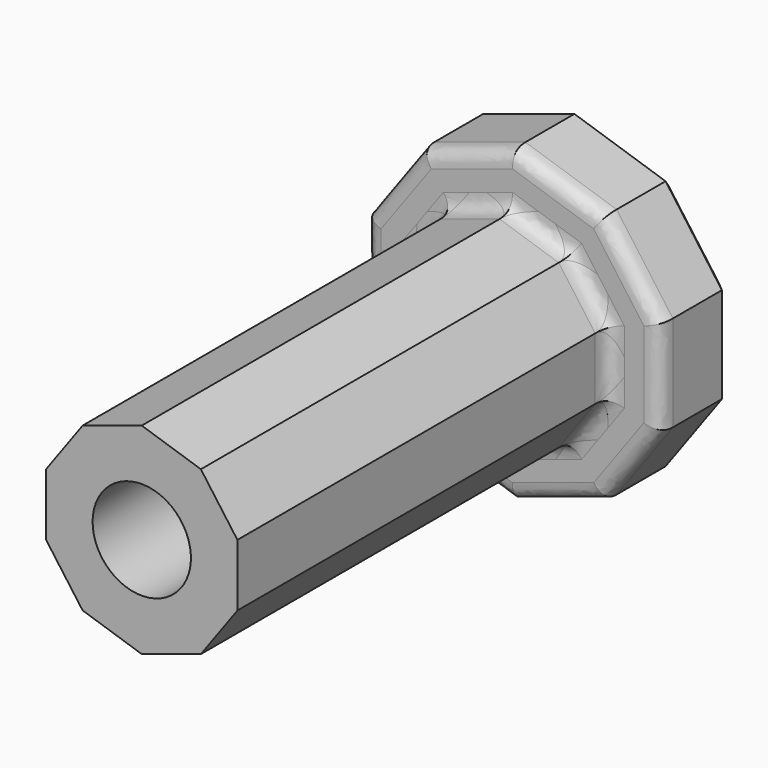
from build123d import *

# Parameters (mm, degrees)
F1_DEPTH      = 76.2
F3_DEPTH      = 6.985
F4_T4_DEPTH   = 21.3495807372
F4_T10_DEPTH  = 21.3495807372
F4_T16_DEPTH  = 21.3495807372
F4_T22_DEPTH  = 21.3495807372
F4_T28_DEPTH  = 21.3495807372
F4_T34_DEPTH  = 21.3495807372
F4_T40_DEPTH  = 21.3495807372
F4_T46_DEPTH  = 21.3495807372
F4_T52_DEPTH  = 21.3495807372
F4_T58_DEPTH  = 21.3495807372
F4_T65_DEPTH  = 21.3495807372
F4_T69_DEPTH  = 21.3495807372
F4_T76_DEPTH  = 21.3495807372
F4_T80_DEPTH  = 21.3495807372
F4_T87_DEPTH  = 21.3495807372
F4_T91_DEPTH  = 21.3495807372
F4_T98_DEPTH  = 21.3495807372
F4_T102_DEPTH = 21.3495807372
F4_T109_DEPTH = 21.3495807372
F4_T113_DEPTH = 21.3495807372
F4_T120_DEPTH = 21.3495807372
F4_T124_DEPTH = 21.3495807372
F4_T131_DEPTH = 21.3495807372
F4_T135_DEPTH = 21.3495807372
F4_T142_DEPTH = 21.3495807372
F4_T146_DEPTH = 21.3495807372
F4_T153_DEPTH = 21.3495807372
F4_T157_DEPTH = 21.3495807372
F4_T164_DEPTH = 21.3495807372
F4_T168_DEPTH = 21.3495807372
F4_T171_DEPTH = 26.3812242456
F4_T173_DEPTH = 26.3812242456
F4_T175_DEPTH = 26.3812242456
F4_T177_DEPTH = 26.3812242456
F4_T179_DEPTH = 26.3812242456
F4_T181_DEPTH = 26.3812242456
F4_T183_DEPTH = 26.3812242456
F4_T185_DEPTH = 26.3812242456
F4_T187_DEPTH = 26.3812242456
F5_SIZE       = 2.413
F7_D          = 14.68374


# Not quite as in the source:
# - a fillet or chamfer that OpenCascade refuses, or shapes differently, is made with other operations: its cross-section is extruded or revolved along the edge and cut away or added


with BuildPart() as f1:
    # F0 (on Front) → F1 (new body)
    with BuildSketch(Plane.XZ):
        Polygon((-14.2875006422, 4.6422903686), (-14.2875006422, -4.6422903686), (-8.8301610112, -12.1536739707), (0, -15.0227672041), (8.8301610112, -12.1536739707), (14.2875006422, -4.6422903686), (14.2875006422, 4.6422903686), (8.8301610112, 12.1536739707), (0, 15.0227672041), (-8.8301610112, 12.1536739707), align=None)
    extrude(amount=F1_DEPTH)

    # F2 (on Front) → F3 (join, symmetric)
    with BuildSketch(Plane.XZ):
        Polygon((-22.0304038376, 7.1581121228), (-22.0304038376, -7.1581121228), (-13.6155383575, -18.7401808327), (0, -23.1641374199), (13.6155383575, -18.7401808327), (22.0304038376, -7.1581121228), (22.0304038376, 7.1581121228), (13.6155383575, 18.7401808327), (0, 23.1641374199), (-13.6155383575, 18.7401808327), align=None)
    extrude(amount=F3_DEPTH, both=True)

    # F4: fillet of radius 2.413 on 20 edges, made by hand


with BuildPart() as f4_tool2:
    # F4_s3 → F4_t4 (new body)
    with BuildSketch(Plane(origin=(10.1523289401, 0, 3.2986916353), x_dir=(0, 1, 0), z_dir=(-0.9510565163, 0, -0.3090169944))):
        with BuildLine():
            add(Edge.make_bspline(
                [(-9.398, -14.2875006422), (-6.985, -14.2875006422), (-6.985, -16.7005006422)],
                knots=[0, 0, 0, 1, 1, 1], degree=2, weights=[1, 1, 1]))
            Line((-6.985, -16.7005006422), (-6.985, -14.2875006422))
            Line((-6.985, -14.2875006422), (-9.398, -14.2875006422))
        make_face()
    extrude(amount=F4_T4_DEPTH)

    split(bisect_by=Plane(origin=(-11.5588308267, 0, 8.3979821696), x_dir=(0, 1, 0), z_dir=(0.8090169944, 0, -0.5877852523)), keep=Keep.TOP)

    split(bisect_by=Plane(origin=(4.4150805056, 0, 13.5882205874), x_dir=(0, 1, 0), z_dir=(-0.3090169944, 0, -0.9510565163)), keep=Keep.TOP)


with BuildPart() as f1_1:
    add(f1.part)

    # F4_t1: union F4_tool2
    add(f4_tool2.part)


with BuildPart() as f4_tool8:
    # F4_s9 → F4_t10 (new body)
    with BuildSketch(Plane(origin=(6.27448435, 0, 8.6360868196), x_dir=(0, 1, 0), z_dir=(-0.5877852523, 0, -0.8090169944))):
        with BuildLine():
            add(Edge.make_bspline(
                [(-6.985, -16.7005006422), (-6.985, -14.2875006422), (-9.398, -14.2875006422)],
                knots=[0, 0, 0, 1, 1, 1], degree=2, weights=[1, 1, 1]))
            Line((-9.398, -14.2875006422), (-6.985, -14.2875006422))
            Line((-6.985, -14.2875006422), (-6.985, -16.7005006422))
        make_face()
    extrude(amount=F4_T10_DEPTH)

    split(bisect_by=Plane(origin=(-4.4150805056, 0, 13.5882205874), x_dir=(0, 1, 0), z_dir=(0.3090169944, 0, -0.9510565163)), keep=Keep.TOP)

    split(bisect_by=Plane.YZ.offset(-14.2875006422), keep=Keep.TOP)


with BuildPart() as f1_2:
    add(f1_1.part)

    # F4_t7: union F4_tool8
    add(f4_tool8.part)


with BuildPart() as f4_tool14:
    # F4_s15 → F4_t16 (new body)
    with BuildSketch(Plane.XY.offset(10.6747903686)):
        with BuildLine():
            add(Edge.make_bspline(
                [(-16.7005006422, -6.985), (-14.2875006422, -6.985), (-14.2875006422, -9.398)],
                knots=[0, 0, 0, 1, 1, 1], degree=2, weights=[1, 1, 1]))
            Line((-14.2875006422, -9.398), (-14.2875006422, -6.985))
            Line((-14.2875006422, -6.985), (-16.7005006422, -6.985))
        make_face()
    extrude(amount=-F4_T16_DEPTH)

    split(bisect_by=Plane(origin=(-11.5588308267, 0, 8.3979821696), x_dir=(0, 1, 0), z_dir=(0.8090169944, 0, -0.5877852523)), keep=Keep.TOP)

    split(bisect_by=Plane(origin=(-11.5588308267, 0, -8.3979821696), x_dir=(0, 1, 0), z_dir=(0.8090169944, 0, 0.5877852523)), keep=Keep.TOP)


with BuildPart() as f1_3:
    add(f1_2.part)

    # F4_t13: union F4_tool14
    add(f4_tool14.part)


with BuildPart() as f4_tool20:
    # F4_s21 → F4_t22 (new body)
    with BuildSketch(Plane(origin=(-6.27448435, 0, 8.6360868196), x_dir=(0, 1, 0), z_dir=(0.5877852523, 0, -0.8090169944))):
        with BuildLine():
            add(Edge.make_bspline(
                [(-6.985, -16.7005006422), (-6.985, -14.2875006422), (-9.398, -14.2875006422)],
                knots=[0, 0, 0, 1, 1, 1], degree=2, weights=[1, 1, 1]))
            Line((-9.398, -14.2875006422), (-6.985, -14.2875006422))
            Line((-6.985, -14.2875006422), (-6.985, -16.7005006422))
        make_face()
    extrude(amount=F4_T22_DEPTH)

    split(bisect_by=Plane.YZ.offset(-14.2875006422), keep=Keep.TOP)

    split(bisect_by=Plane(origin=(-4.4150805056, 0, -13.5882205874), x_dir=(0, 1, 0), z_dir=(0.3090169944, 0, 0.9510565163)), keep=Keep.TOP)


with BuildPart() as f1_4:
    add(f1_3.part)

    # F4_t19: union F4_tool20
    add(f4_tool20.part)


with BuildPart() as f4_tool26:
    # F4_s27 → F4_t28 (new body)
    with BuildSketch(Plane(origin=(-10.1523289401, 0, 3.2986916353), x_dir=(0, 1, 0), z_dir=(0.9510565163, 0, -0.3090169944))):
        with BuildLine():
            add(Edge.make_bspline(
                [(-6.985, -16.7005006422), (-6.985, -14.2875006422), (-9.398, -14.2875006422)],
                knots=[0, 0, 0, 1, 1, 1], degree=2, weights=[1, 1, 1]))
            Line((-9.398, -14.2875006422), (-6.985, -14.2875006422))
            Line((-6.985, -14.2875006422), (-6.985, -16.7005006422))
        make_face()
    extrude(amount=F4_T28_DEPTH)

    split(bisect_by=Plane(origin=(-11.5588308267, 0, -8.3979821696), x_dir=(0, 1, 0), z_dir=(0.8090169944, 0, 0.5877852523)), keep=Keep.TOP)

    split(bisect_by=Plane(origin=(4.4150805056, 0, -13.5882205874), x_dir=(0, 1, 0), z_dir=(-0.3090169944, 0, 0.9510565163)), keep=Keep.TOP)


with BuildPart() as f1_5:
    add(f1_4.part)

    # F4_t25: union F4_tool26
    add(f4_tool26.part)


with BuildPart() as f4_tool32:
    # F4_s33 → F4_t34 (new body)
    with BuildSketch(Plane(origin=(-10.1523289401, 0, -3.2986916353), x_dir=(0, 1, 0), z_dir=(0.9510565163, 0, 0.3090169944))):
        with BuildLine():
            add(Edge.make_bspline(
                [(-6.985, -16.7005006422), (-6.985, -14.2875006422), (-9.398, -14.2875006422)],
                knots=[0, 0, 0, 1, 1, 1], degree=2, weights=[1, 1, 1]))
            Line((-9.398, -14.2875006422), (-6.985, -14.2875006422))
            Line((-6.985, -14.2875006422), (-6.985, -16.7005006422))
        make_face()
    extrude(amount=F4_T34_DEPTH)

    split(bisect_by=Plane(origin=(-4.4150805056, 0, -13.5882205874), x_dir=(0, 1, 0), z_dir=(0.3090169944, 0, 0.9510565163)), keep=Keep.TOP)

    split(bisect_by=Plane(origin=(11.5588308267, 0, -8.3979821696), x_dir=(0, 1, 0), z_dir=(-0.8090169944, 0, 0.5877852523)), keep=Keep.TOP)


with BuildPart() as f1_6:
    add(f1_5.part)

    # F4_t31: union F4_tool32
    add(f4_tool32.part)


with BuildPart() as f4_tool38:
    # F4_s39 → F4_t40 (new body)
    with BuildSketch(Plane(origin=(-6.27448435, 0, -8.6360868196), x_dir=(0, 1, 0), z_dir=(0.5877852523, 0, 0.8090169944))):
        with BuildLine():
            add(Edge.make_bspline(
                [(-6.985, -16.7005006422), (-6.985, -14.2875006422), (-9.398, -14.2875006422)],
                knots=[0, 0, 0, 1, 1, 1], degree=2, weights=[1, 1, 1]))
            Line((-9.398, -14.2875006422), (-6.985, -14.2875006422))
            Line((-6.985, -14.2875006422), (-6.985, -16.7005006422))
        make_face()
    extrude(amount=F4_T40_DEPTH)

    split(bisect_by=Plane(origin=(4.4150805056, 0, -13.5882205874), x_dir=(0, 1, 0), z_dir=(-0.3090169944, 0, 0.9510565163)), keep=Keep.TOP)

    split(bisect_by=Plane.YZ.offset(14.2875006422), keep=Keep.BOTTOM)


with BuildPart() as f1_7:
    add(f1_6.part)

    # F4_t37: union F4_tool38
    add(f4_tool38.part)


with BuildPart() as f4_tool44:
    # F4_s45 → F4_t46 (new body)
    with BuildSketch(Plane.XY.offset(-10.6747903686)):
        with BuildLine():
            add(Edge.make_bspline(
                [(16.7005006422, -6.985), (14.2875006422, -6.985), (14.2875006422, -9.398)],
                knots=[0, 0, 0, 1, 1, 1], degree=2, weights=[1, 1, 1]))
            Line((14.2875006422, -9.398), (14.2875006422, -6.985))
            Line((14.2875006422, -6.985), (16.7005006422, -6.985))
        make_face()
    extrude(amount=F4_T46_DEPTH)

    split(bisect_by=Plane(origin=(11.5588308267, 0, -8.3979821696), x_dir=(0, 1, 0), z_dir=(-0.8090169944, 0, 0.5877852523)), keep=Keep.TOP)

    split(bisect_by=Plane(origin=(11.5588308267, 0, 8.3979821696), x_dir=(0, 1, 0), z_dir=(-0.8090169944, 0, -0.5877852523)), keep=Keep.TOP)


with BuildPart() as f1_8:
    add(f1_7.part)

    # F4_t43: union F4_tool44
    add(f4_tool44.part)


with BuildPart() as f4_tool50:
    # F4_s51 → F4_t52 (new body)
    with BuildSketch(Plane(origin=(6.27448435, 0, -8.6360868196), x_dir=(0, 1, 0), z_dir=(-0.5877852523, 0, 0.8090169944))):
        with BuildLine():
            add(Edge.make_bspline(
                [(-6.985, -16.7005006422), (-6.985, -14.2875006422), (-9.398, -14.2875006422)],
                knots=[0, 0, 0, 1, 1, 1], degree=2, weights=[1, 1, 1]))
            Line((-9.398, -14.2875006422), (-6.985, -14.2875006422))
            Line((-6.985, -14.2875006422), (-6.985, -16.7005006422))
        make_face()
    extrude(amount=F4_T52_DEPTH)

    split(bisect_by=Plane(origin=(4.4150805056, 0, 13.5882205874), x_dir=(0, 1, 0), z_dir=(-0.3090169944, 0, -0.9510565163)), keep=Keep.TOP)

    split(bisect_by=Plane.YZ.offset(14.2875006422), keep=Keep.BOTTOM)


with BuildPart() as f1_9:
    add(f1_8.part)

    # F4_t49: union F4_tool50
    add(f4_tool50.part)


with BuildPart() as f4_tool56:
    # F4_s57 → F4_t58 (new body)
    with BuildSketch(Plane(origin=(10.1523289401, 0, -3.2986916353), x_dir=(0, 1, 0), z_dir=(-0.9510565163, 0, 0.3090169944))):
        with BuildLine():
            add(Edge.make_bspline(
                [(-6.985, -16.7005006422), (-6.985, -14.2875006422), (-9.398, -14.2875006422)],
                knots=[0, 0, 0, 1, 1, 1], degree=2, weights=[1, 1, 1]))
            Line((-9.398, -14.2875006422), (-6.985, -14.2875006422))
            Line((-6.985, -14.2875006422), (-6.985, -16.7005006422))
        make_face()
    extrude(amount=F4_T58_DEPTH)

    split(bisect_by=Plane(origin=(-4.4150805056, 0, 13.5882205874), x_dir=(0, 1, 0), z_dir=(0.3090169944, 0, -0.9510565163)), keep=Keep.TOP)

    split(bisect_by=Plane(origin=(11.5588308267, 0, 8.3979821696), x_dir=(0, 1, 0), z_dir=(-0.8090169944, 0, -0.5877852523)), keep=Keep.TOP)


with BuildPart() as f1_10:
    add(f1_9.part)

    # F4_t55: union F4_tool56
    add(f4_tool56.part)


with BuildPart() as f4_tool63:
    # F4_s64 → F4_t65 (new body)
    with BuildSketch(Plane(origin=(10.1523289401, 0, 3.2986916353), x_dir=(0, 1, 0), z_dir=(-0.9510565163, 0, -0.3090169944))):
        with BuildLine():
            add(Edge.make_bspline(
                [(-9.398, -14.2875006422), (-6.985, -14.2875006422), (-6.985, -16.7005006422)],
                knots=[0, 0, 0, 1, 1, 1], degree=2, weights=[1, 1, 1]))
            Line((-6.985, -16.7005006422), (-6.985, -14.2875006422))
            Line((-6.985, -14.2875006422), (-9.398, -14.2875006422))
        make_face()
    extrude(amount=F4_T65_DEPTH)

    split(bisect_by=Plane(origin=(4.4150805056, 0, 13.5882205874), x_dir=(0, 1, 0), z_dir=(0.3090169944, 0, 0.9510565163)), keep=Keep.TOP)


with BuildPart() as f4_tool67:
    # F4_s68 → F4_t69 (new body)
    with BuildSketch(Plane(origin=(10.1523289401, 0, -3.2986916353), x_dir=(0, 1, 0), z_dir=(-0.9510565163, 0, 0.3090169944))):
        with BuildLine():
            add(Edge.make_bspline(
                [(-6.985, -16.7005006422), (-6.985, -14.2875006422), (-9.398, -14.2875006422)],
                knots=[0, 0, 0, 1, 1, 1], degree=2, weights=[1, 1, 1]))
            Line((-9.398, -14.2875006422), (-6.985, -14.2875006422))
            Line((-6.985, -14.2875006422), (-6.985, -16.7005006422))
        make_face()
    extrude(amount=F4_T69_DEPTH)

    split(bisect_by=Plane(origin=(-4.4150805056, 0, 13.5882205874), x_dir=(0, 1, 0), z_dir=(-0.3090169944, 0, 0.9510565163)), keep=Keep.TOP)


with BuildPart() as f4_tool63_1:
    add(f4_tool63.part)

    # F4_t71: intersect F4_tool67
    add(f4_tool67.part, mode=Mode.INTERSECT)


with BuildPart() as f1_11:
    add(f1_10.part)

    # F4_t61: union F4_tool63
    add(f4_tool63_1.part)


with BuildPart() as f4_tool74:
    # F4_s75 → F4_t76 (new body)
    with BuildSketch(Plane(origin=(10.1523289401, 0, 3.2986916353), x_dir=(0, 1, 0), z_dir=(-0.9510565163, 0, -0.3090169944))):
        with BuildLine():
            add(Edge.make_bspline(
                [(-9.398, -14.2875006422), (-6.985, -14.2875006422), (-6.985, -16.7005006422)],
                knots=[0, 0, 0, 1, 1, 1], degree=2, weights=[1, 1, 1]))
            Line((-6.985, -16.7005006422), (-6.985, -14.2875006422))
            Line((-6.985, -14.2875006422), (-9.398, -14.2875006422))
        make_face()
    extrude(amount=F4_T76_DEPTH)

    split(bisect_by=Plane(origin=(-11.5588308267, 0, 8.3979821696), x_dir=(0, 1, 0), z_dir=(-0.8090169944, 0, 0.5877852523)), keep=Keep.TOP)


with BuildPart() as f4_tool78:
    # F4_s79 → F4_t80 (new body)
    with BuildSketch(Plane(origin=(6.27448435, 0, 8.6360868196), x_dir=(0, 1, 0), z_dir=(-0.5877852523, 0, -0.8090169944))):
        with BuildLine():
            add(Edge.make_bspline(
                [(-6.985, -16.7005006422), (-6.985, -14.2875006422), (-9.398, -14.2875006422)],
                knots=[0, 0, 0, 1, 1, 1], degree=2, weights=[1, 1, 1]))
            Line((-9.398, -14.2875006422), (-6.985, -14.2875006422))
            Line((-6.985, -14.2875006422), (-6.985, -16.7005006422))
        make_face()
    extrude(amount=F4_T80_DEPTH)

    split(bisect_by=Plane(origin=(-4.4150805056, 0, 13.5882205874), x_dir=(0, 1, 0), z_dir=(-0.3090169944, 0, 0.9510565163)), keep=Keep.TOP)


with BuildPart() as f4_tool74_1:
    add(f4_tool74.part)

    # F4_t82: intersect F4_tool78
    add(f4_tool78.part, mode=Mode.INTERSECT)


with BuildPart() as f1_12:
    add(f1_11.part)

    # F4_t72: union F4_tool74
    add(f4_tool74_1.part)


with BuildPart() as f4_tool85:
    # F4_s86 → F4_t87 (new body)
    with BuildSketch(Plane(origin=(6.27448435, 0, 8.6360868196), x_dir=(0, 1, 0), z_dir=(-0.5877852523, 0, -0.8090169944))):
        with BuildLine():
            add(Edge.make_bspline(
                [(-6.985, -16.7005006422), (-6.985, -14.2875006422), (-9.398, -14.2875006422)],
                knots=[0, 0, 0, 1, 1, 1], degree=2, weights=[1, 1, 1]))
            Line((-9.398, -14.2875006422), (-6.985, -14.2875006422))
            Line((-6.985, -14.2875006422), (-6.985, -16.7005006422))
        make_face()
    extrude(amount=F4_T87_DEPTH)

    split(bisect_by=Plane.YZ.offset(-14.2875006422), keep=Keep.BOTTOM)


with BuildPart() as f4_tool89:
    # F4_s90 → F4_t91 (new body)
    with BuildSketch(Plane.XY.offset(10.6747903686)):
        with BuildLine():
            add(Edge.make_bspline(
                [(-16.7005006422, -6.985), (-14.2875006422, -6.985), (-14.2875006422, -9.398)],
                knots=[0, 0, 0, 1, 1, 1], degree=2, weights=[1, 1, 1]))
            Line((-14.2875006422, -9.398), (-14.2875006422, -6.985))
            Line((-14.2875006422, -6.985), (-16.7005006422, -6.985))
        make_face()
    extrude(amount=-F4_T91_DEPTH)

    split(bisect_by=Plane(origin=(-11.5588308267, 0, 8.3979821696), x_dir=(0, 1, 0), z_dir=(-0.8090169944, 0, 0.5877852523)), keep=Keep.TOP)


with BuildPart() as f4_tool85_1:
    add(f4_tool85.part)

    # F4_t93: intersect F4_tool89
    add(f4_tool89.part, mode=Mode.INTERSECT)


with BuildPart() as f1_13:
    add(f1_12.part)

    # F4_t83: union F4_tool85
    add(f4_tool85_1.part)


with BuildPart() as f4_tool96:
    # F4_s97 → F4_t98 (new body)
    with BuildSketch(Plane.XY.offset(10.6747903686)):
        with BuildLine():
            add(Edge.make_bspline(
                [(-16.7005006422, -6.985), (-14.2875006422, -6.985), (-14.2875006422, -9.398)],
                knots=[0, 0, 0, 1, 1, 1], degree=2, weights=[1, 1, 1]))
            Line((-14.2875006422, -9.398), (-14.2875006422, -6.985))
            Line((-14.2875006422, -6.985), (-16.7005006422, -6.985))
        make_face()
    extrude(amount=-F4_T98_DEPTH)

    split(bisect_by=Plane(origin=(-11.5588308267, 0, -8.3979821696), x_dir=(0, 1, 0), z_dir=(-0.8090169944, 0, -0.5877852523)), keep=Keep.TOP)


with BuildPart() as f4_tool100:
    # F4_s101 → F4_t102 (new body)
    with BuildSketch(Plane(origin=(-6.27448435, 0, 8.6360868196), x_dir=(0, 1, 0), z_dir=(0.5877852523, 0, -0.8090169944))):
        with BuildLine():
            add(Edge.make_bspline(
                [(-6.985, -16.7005006422), (-6.985, -14.2875006422), (-9.398, -14.2875006422)],
                knots=[0, 0, 0, 1, 1, 1], degree=2, weights=[1, 1, 1]))
            Line((-9.398, -14.2875006422), (-6.985, -14.2875006422))
            Line((-6.985, -14.2875006422), (-6.985, -16.7005006422))
        make_face()
    extrude(amount=F4_T102_DEPTH)

    split(bisect_by=Plane.YZ.offset(-14.2875006422), keep=Keep.BOTTOM)


with BuildPart() as f4_tool96_1:
    add(f4_tool96.part)

    # F4_t104: intersect F4_tool100
    add(f4_tool100.part, mode=Mode.INTERSECT)


with BuildPart() as f1_14:
    add(f1_13.part)

    # F4_t94: union F4_tool96
    add(f4_tool96_1.part)


with BuildPart() as f4_tool107:
    # F4_s108 → F4_t109 (new body)
    with BuildSketch(Plane(origin=(-6.27448435, 0, 8.6360868196), x_dir=(0, 1, 0), z_dir=(0.5877852523, 0, -0.8090169944))):
        with BuildLine():
            add(Edge.make_bspline(
                [(-6.985, -16.7005006422), (-6.985, -14.2875006422), (-9.398, -14.2875006422)],
                knots=[0, 0, 0, 1, 1, 1], degree=2, weights=[1, 1, 1]))
            Line((-9.398, -14.2875006422), (-6.985, -14.2875006422))
            Line((-6.985, -14.2875006422), (-6.985, -16.7005006422))
        make_face()
    extrude(amount=F4_T109_DEPTH)

    split(bisect_by=Plane(origin=(-4.4150805056, 0, -13.5882205874), x_dir=(0, 1, 0), z_dir=(-0.3090169944, 0, -0.9510565163)), keep=Keep.TOP)


with BuildPart() as f4_tool111:
    # F4_s112 → F4_t113 (new body)
    with BuildSketch(Plane(origin=(-10.1523289401, 0, 3.2986916353), x_dir=(0, 1, 0), z_dir=(0.9510565163, 0, -0.3090169944))):
        with BuildLine():
            add(Edge.make_bspline(
                [(-6.985, -16.7005006422), (-6.985, -14.2875006422), (-9.398, -14.2875006422)],
                knots=[0, 0, 0, 1, 1, 1], degree=2, weights=[1, 1, 1]))
            Line((-9.398, -14.2875006422), (-6.985, -14.2875006422))
            Line((-6.985, -14.2875006422), (-6.985, -16.7005006422))
        make_face()
    extrude(amount=F4_T113_DEPTH)

    split(bisect_by=Plane(origin=(-11.5588308267, 0, -8.3979821696), x_dir=(0, 1, 0), z_dir=(-0.8090169944, 0, -0.5877852523)), keep=Keep.TOP)


with BuildPart() as f4_tool107_1:
    add(f4_tool107.part)

    # F4_t115: intersect F4_tool111
    add(f4_tool111.part, mode=Mode.INTERSECT)


with BuildPart() as f1_15:
    add(f1_14.part)

    # F4_t105: union F4_tool107
    add(f4_tool107_1.part)


with BuildPart() as f4_tool118:
    # F4_s119 → F4_t120 (new body)
    with BuildSketch(Plane(origin=(-10.1523289401, 0, 3.2986916353), x_dir=(0, 1, 0), z_dir=(0.9510565163, 0, -0.3090169944))):
        with BuildLine():
            add(Edge.make_bspline(
                [(-6.985, -16.7005006422), (-6.985, -14.2875006422), (-9.398, -14.2875006422)],
                knots=[0, 0, 0, 1, 1, 1], degree=2, weights=[1, 1, 1]))
            Line((-9.398, -14.2875006422), (-6.985, -14.2875006422))
            Line((-6.985, -14.2875006422), (-6.985, -16.7005006422))
        make_face()
    extrude(amount=F4_T120_DEPTH)

    split(bisect_by=Plane(origin=(4.4150805056, 0, -13.5882205874), x_dir=(0, 1, 0), z_dir=(0.3090169944, 0, -0.9510565163)), keep=Keep.TOP)


with BuildPart() as f4_tool122:
    # F4_s123 → F4_t124 (new body)
    with BuildSketch(Plane(origin=(-10.1523289401, 0, -3.2986916353), x_dir=(0, 1, 0), z_dir=(0.9510565163, 0, 0.3090169944))):
        with BuildLine():
            add(Edge.make_bspline(
                [(-6.985, -16.7005006422), (-6.985, -14.2875006422), (-9.398, -14.2875006422)],
                knots=[0, 0, 0, 1, 1, 1], degree=2, weights=[1, 1, 1]))
            Line((-9.398, -14.2875006422), (-6.985, -14.2875006422))
            Line((-6.985, -14.2875006422), (-6.985, -16.7005006422))
        make_face()
    extrude(amount=F4_T124_DEPTH)

    split(bisect_by=Plane(origin=(-4.4150805056, 0, -13.5882205874), x_dir=(0, 1, 0), z_dir=(-0.3090169944, 0, -0.9510565163)), keep=Keep.TOP)


with BuildPart() as f4_tool118_1:
    add(f4_tool118.part)

    # F4_t126: intersect F4_tool122
    add(f4_tool122.part, mode=Mode.INTERSECT)


with BuildPart() as f1_16:
    add(f1_15.part)

    # F4_t116: union F4_tool118
    add(f4_tool118_1.part)


with BuildPart() as f4_tool129:
    # F4_s130 → F4_t131 (new body)
    with BuildSketch(Plane(origin=(-10.1523289401, 0, -3.2986916353), x_dir=(0, 1, 0), z_dir=(0.9510565163, 0, 0.3090169944))):
        with BuildLine():
            add(Edge.make_bspline(
                [(-6.985, -16.7005006422), (-6.985, -14.2875006422), (-9.398, -14.2875006422)],
                knots=[0, 0, 0, 1, 1, 1], degree=2, weights=[1, 1, 1]))
            Line((-9.398, -14.2875006422), (-6.985, -14.2875006422))
            Line((-6.985, -14.2875006422), (-6.985, -16.7005006422))
        make_face()
    extrude(amount=F4_T131_DEPTH)

    split(bisect_by=Plane(origin=(11.5588308267, 0, -8.3979821696), x_dir=(0, 1, 0), z_dir=(0.8090169944, 0, -0.5877852523)), keep=Keep.TOP)


with BuildPart() as f4_tool133:
    # F4_s134 → F4_t135 (new body)
    with BuildSketch(Plane(origin=(-6.27448435, 0, -8.6360868196), x_dir=(0, 1, 0), z_dir=(0.5877852523, 0, 0.8090169944))):
        with BuildLine():
            add(Edge.make_bspline(
                [(-6.985, -16.7005006422), (-6.985, -14.2875006422), (-9.398, -14.2875006422)],
                knots=[0, 0, 0, 1, 1, 1], degree=2, weights=[1, 1, 1]))
            Line((-9.398, -14.2875006422), (-6.985, -14.2875006422))
            Line((-6.985, -14.2875006422), (-6.985, -16.7005006422))
        make_face()
    extrude(amount=F4_T135_DEPTH)

    split(bisect_by=Plane(origin=(4.4150805056, 0, -13.5882205874), x_dir=(0, 1, 0), z_dir=(0.3090169944, 0, -0.9510565163)), keep=Keep.TOP)


with BuildPart() as f4_tool129_1:
    add(f4_tool129.part)

    # F4_t137: intersect F4_tool133
    add(f4_tool133.part, mode=Mode.INTERSECT)


with BuildPart() as f1_17:
    add(f1_16.part)

    # F4_t127: union F4_tool129
    add(f4_tool129_1.part)


with BuildPart() as f4_tool140:
    # F4_s141 → F4_t142 (new body)
    with BuildSketch(Plane(origin=(-6.27448435, 0, -8.6360868196), x_dir=(0, 1, 0), z_dir=(0.5877852523, 0, 0.8090169944))):
        with BuildLine():
            add(Edge.make_bspline(
                [(-6.985, -16.7005006422), (-6.985, -14.2875006422), (-9.398, -14.2875006422)],
                knots=[0, 0, 0, 1, 1, 1], degree=2, weights=[1, 1, 1]))
            Line((-9.398, -14.2875006422), (-6.985, -14.2875006422))
            Line((-6.985, -14.2875006422), (-6.985, -16.7005006422))
        make_face()
    extrude(amount=F4_T142_DEPTH)

    split(bisect_by=Plane.YZ.offset(14.2875006422), keep=Keep.TOP)


with BuildPart() as f4_tool144:
    # F4_s145 → F4_t146 (new body)
    with BuildSketch(Plane.XY.offset(-10.6747903686)):
        with BuildLine():
            add(Edge.make_bspline(
                [(16.7005006422, -6.985), (14.2875006422, -6.985), (14.2875006422, -9.398)],
                knots=[0, 0, 0, 1, 1, 1], degree=2, weights=[1, 1, 1]))
            Line((14.2875006422, -9.398), (14.2875006422, -6.985))
            Line((14.2875006422, -6.985), (16.7005006422, -6.985))
        make_face()
    extrude(amount=F4_T146_DEPTH)

    split(bisect_by=Plane(origin=(11.5588308267, 0, -8.3979821696), x_dir=(0, 1, 0), z_dir=(0.8090169944, 0, -0.5877852523)), keep=Keep.TOP)


with BuildPart() as f4_tool140_1:
    add(f4_tool140.part)

    # F4_t148: intersect F4_tool144
    add(f4_tool144.part, mode=Mode.INTERSECT)


with BuildPart() as f1_18:
    add(f1_17.part)

    # F4_t138: union F4_tool140
    add(f4_tool140_1.part)


with BuildPart() as f4_tool151:
    # F4_s152 → F4_t153 (new body)
    with BuildSketch(Plane.XY.offset(-10.6747903686)):
        with BuildLine():
            add(Edge.make_bspline(
                [(16.7005006422, -6.985), (14.2875006422, -6.985), (14.2875006422, -9.398)],
                knots=[0, 0, 0, 1, 1, 1], degree=2, weights=[1, 1, 1]))
            Line((14.2875006422, -9.398), (14.2875006422, -6.985))
            Line((14.2875006422, -6.985), (16.7005006422, -6.985))
        make_face()
    extrude(amount=F4_T153_DEPTH)

    split(bisect_by=Plane(origin=(11.5588308267, 0, 8.3979821696), x_dir=(0, 1, 0), z_dir=(0.8090169944, 0, 0.5877852523)), keep=Keep.TOP)


with BuildPart() as f4_tool155:
    # F4_s156 → F4_t157 (new body)
    with BuildSketch(Plane(origin=(6.27448435, 0, -8.6360868196), x_dir=(0, 1, 0), z_dir=(-0.5877852523, 0, 0.8090169944))):
        with BuildLine():
            add(Edge.make_bspline(
                [(-6.985, -16.7005006422), (-6.985, -14.2875006422), (-9.398, -14.2875006422)],
                knots=[0, 0, 0, 1, 1, 1], degree=2, weights=[1, 1, 1]))
            Line((-9.398, -14.2875006422), (-6.985, -14.2875006422))
            Line((-6.985, -14.2875006422), (-6.985, -16.7005006422))
        make_face()
    extrude(amount=F4_T157_DEPTH)

    split(bisect_by=Plane.YZ.offset(14.2875006422), keep=Keep.TOP)


with BuildPart() as f4_tool151_1:
    add(f4_tool151.part)

    # F4_t159: intersect F4_tool155
    add(f4_tool155.part, mode=Mode.INTERSECT)


with BuildPart() as f1_19:
    add(f1_18.part)

    # F4_t149: union F4_tool151
    add(f4_tool151_1.part)


with BuildPart() as f4_tool162:
    # F4_s163 → F4_t164 (new body)
    with BuildSketch(Plane(origin=(6.27448435, 0, -8.6360868196), x_dir=(0, 1, 0), z_dir=(-0.5877852523, 0, 0.8090169944))):
        with BuildLine():
            add(Edge.make_bspline(
                [(-6.985, -16.7005006422), (-6.985, -14.2875006422), (-9.398, -14.2875006422)],
                knots=[0, 0, 0, 1, 1, 1], degree=2, weights=[1, 1, 1]))
            Line((-9.398, -14.2875006422), (-6.985, -14.2875006422))
            Line((-6.985, -14.2875006422), (-6.985, -16.7005006422))
        make_face()
    extrude(amount=F4_T164_DEPTH)

    split(bisect_by=Plane(origin=(4.4150805056, 0, 13.5882205874), x_dir=(0, 1, 0), z_dir=(0.3090169944, 0, 0.9510565163)), keep=Keep.TOP)


with BuildPart() as f4_tool166:
    # F4_s167 → F4_t168 (new body)
    with BuildSketch(Plane(origin=(10.1523289401, 0, -3.2986916353), x_dir=(0, 1, 0), z_dir=(-0.9510565163, 0, 0.3090169944))):
        with BuildLine():
            add(Edge.make_bspline(
                [(-6.985, -16.7005006422), (-6.985, -14.2875006422), (-9.398, -14.2875006422)],
                knots=[0, 0, 0, 1, 1, 1], degree=2, weights=[1, 1, 1]))
            Line((-9.398, -14.2875006422), (-6.985, -14.2875006422))
            Line((-6.985, -14.2875006422), (-6.985, -16.7005006422))
        make_face()
    extrude(amount=F4_T168_DEPTH)

    split(bisect_by=Plane(origin=(11.5588308267, 0, 8.3979821696), x_dir=(0, 1, 0), z_dir=(0.8090169944, 0, 0.5877852523)), keep=Keep.TOP)


with BuildPart() as f4_tool162_1:
    add(f4_tool162.part)

    # F4_t170: intersect F4_tool166
    add(f4_tool166.part, mode=Mode.INTERSECT)


with BuildPart() as f1_20:
    add(f1_19.part)

    # F4_t160: union F4_tool162
    add(f4_tool162_1.part)

    # F4_s172 → F4_t171 (cut)
    with BuildSketch(Plane(origin=(7.7532472745, 0, 10.6714293735), x_dir=(0, 1, 0), z_dir=(-0.5877852523, 0, -0.8090169944))):
        with BuildLine():
            add(Edge.make_bspline(
                [(-6.985, -19.6174038376), (-6.985, -22.0304038376), (-4.572, -22.0304038376)],
                knots=[0, 0, 0, 1, 1, 1], degree=2, weights=[1, 1, 1]))
            Line((-4.572, -22.0304038376), (-6.985, -22.0304038376))
            Line((-6.985, -22.0304038376), (-6.985, -19.6174038376))
        make_face()
    extrude(amount=F4_T171_DEPTH, mode=Mode.SUBTRACT)

    # F4_s174 → F4_t173 (cut)
    with BuildSketch(Plane(origin=(12.5450176133, 0, 4.0761233121), x_dir=(0, 1, 0), z_dir=(-0.9510565163, 0, -0.3090169944))):
        with BuildLine():
            add(Edge.make_bspline(
                [(-6.985, -19.6174038376), (-6.985, -22.0304038376), (-4.572, -22.0304038376)],
                knots=[0, 0, 0, 1, 1, 1], degree=2, weights=[1, 1, 1]))
            Line((-4.572, -22.0304038376), (-6.985, -22.0304038376))
            Line((-6.985, -22.0304038376), (-6.985, -19.6174038376))
        make_face()
    extrude(amount=F4_T173_DEPTH, mode=Mode.SUBTRACT)

    # F4_s176 → F4_t175 (cut)
    with BuildSketch(Plane.XY.offset(-13.1906121228)):
        with BuildLine():
            add(Edge.make_bspline(
                [(-19.6174038376, -6.985), (-22.0304038376, -6.985), (-22.0304038376, -4.572)],
                knots=[0, 0, 0, 1, 1, 1], degree=2, weights=[1, 1, 1]))
            Line((-22.0304038376, -4.572), (-22.0304038376, -6.985))
            Line((-22.0304038376, -6.985), (-19.6174038376, -6.985))
        make_face()
        with BuildLine():
            add(Edge.make_bspline(
                [(19.6174038376, -6.985), (22.0304038376, -6.985), (22.0304038376, -4.572)],
                knots=[0, 0, 0, 1, 1, 1], degree=2, weights=[1, 1, 1]))
            Line((22.0304038376, -4.572), (22.0304038376, -6.985))
            Line((22.0304038376, -6.985), (19.6174038376, -6.985))
        make_face()
    extrude(amount=F4_T175_DEPTH, mode=Mode.SUBTRACT)

    # F4_s178 → F4_t177 (cut)
    with BuildSketch(Plane(origin=(12.5450176133, 0, -4.0761233121), x_dir=(0, 1, 0), z_dir=(-0.9510565163, 0, 0.3090169944))):
        with BuildLine():
            add(Edge.make_bspline(
                [(-6.985, -19.6174038376), (-6.985, -22.0304038376), (-4.572, -22.0304038376)],
                knots=[0, 0, 0, 1, 1, 1], degree=2, weights=[1, 1, 1]))
            Line((-4.572, -22.0304038376), (-6.985, -22.0304038376))
            Line((-6.985, -22.0304038376), (-6.985, -19.6174038376))
        make_face()
    extrude(amount=F4_T177_DEPTH, mode=Mode.SUBTRACT)

    # F4_s180 → F4_t179 (cut)
    with BuildSketch(Plane(origin=(-7.7532472745, 0, 10.6714293735), x_dir=(0, 1, 0), z_dir=(0.5877852523, 0, -0.8090169944))):
        with BuildLine():
            add(Edge.make_bspline(
                [(-6.985, -19.6174038376), (-6.985, -22.0304038376), (-4.572, -22.0304038376)],
                knots=[0, 0, 0, 1, 1, 1], degree=2, weights=[1, 1, 1]))
            Line((-4.572, -22.0304038376), (-6.985, -22.0304038376))
            Line((-6.985, -22.0304038376), (-6.985, -19.6174038376))
        make_face()
    extrude(amount=F4_T179_DEPTH, mode=Mode.SUBTRACT)

    # F4_s182 → F4_t181 (cut)
    with BuildSketch(Plane(origin=(7.7532472745, 0, -10.6714293735), x_dir=(0, 1, 0), z_dir=(-0.5877852523, 0, 0.8090169944))):
        with BuildLine():
            add(Edge.make_bspline(
                [(-6.985, -19.6174038376), (-6.985, -22.0304038376), (-4.572, -22.0304038376)],
                knots=[0, 0, 0, 1, 1, 1], degree=2, weights=[1, 1, 1]))
            Line((-4.572, -22.0304038376), (-6.985, -22.0304038376))
            Line((-6.985, -22.0304038376), (-6.985, -19.6174038376))
        make_face()
    extrude(amount=F4_T181_DEPTH, mode=Mode.SUBTRACT)

    # F4_s184 → F4_t183 (cut)
    with BuildSketch(Plane(origin=(-12.5450176133, 0, 4.0761233121), x_dir=(0, 1, 0), z_dir=(0.9510565163, 0, -0.3090169944))):
        with BuildLine():
            add(Edge.make_bspline(
                [(-6.985, -19.6174038376), (-6.985, -22.0304038376), (-4.572, -22.0304038376)],
                knots=[0, 0, 0, 1, 1, 1], degree=2, weights=[1, 1, 1]))
            Line((-4.572, -22.0304038376), (-6.985, -22.0304038376))
            Line((-6.985, -22.0304038376), (-6.985, -19.6174038376))
        make_face()
    extrude(amount=F4_T183_DEPTH, mode=Mode.SUBTRACT)

    # F4_s186 → F4_t185 (cut)
    with BuildSketch(Plane(origin=(-12.5450176133, 0, -4.0761233121), x_dir=(0, 1, 0), z_dir=(0.9510565163, 0, 0.3090169944))):
        with BuildLine():
            add(Edge.make_bspline(
                [(-6.985, -19.6174038376), (-6.985, -22.0304038376), (-4.572, -22.0304038376)],
                knots=[0, 0, 0, 1, 1, 1], degree=2, weights=[1, 1, 1]))
            Line((-4.572, -22.0304038376), (-6.985, -22.0304038376))
            Line((-6.985, -22.0304038376), (-6.985, -19.6174038376))
        make_face()
    extrude(amount=F4_T185_DEPTH, mode=Mode.SUBTRACT)

    # F4_s188 → F4_t187 (cut)
    with BuildSketch(Plane(origin=(-7.7532472745, 0, -10.6714293735), x_dir=(0, 1, 0), z_dir=(0.5877852523, 0, 0.8090169944))):
        with BuildLine():
            add(Edge.make_bspline(
                [(-6.985, -19.6174038376), (-6.985, -22.0304038376), (-4.572, -22.0304038376)],
                knots=[0, 0, 0, 1, 1, 1], degree=2, weights=[1, 1, 1]))
            Line((-4.572, -22.0304038376), (-6.985, -22.0304038376))
            Line((-6.985, -22.0304038376), (-6.985, -19.6174038376))
        make_face()
    extrude(amount=F4_T187_DEPTH, mode=Mode.SUBTRACT)

    # F5
    f5_edges = [f1_20.edges().sort_by_distance(p)[0] for p in [
        (-17.822971, 6.985, 12.949146),
        (-22.030404, 6.985, 0),
        (-17.822971, 6.985, -12.949146),
        (-6.807769, 6.985, -20.952159),
        (6.807769, 6.985, -20.952159),
        (17.822971, 6.985, -12.949146),
        (22.030404, 6.985, 0),
        (17.822971, 6.985, 12.949146),
        (6.807769, 6.985, 20.952159),
        (-6.807769, 6.985, 20.952159),
    ]]
    chamfer(f5_edges, length=F5_SIZE)

    # F7 (through all)
    with Locations(Plane.XZ.offset(76.2)):
        with Locations((0, 0)):
            Hole(F7_D / 2)


solid = f1_20.part
